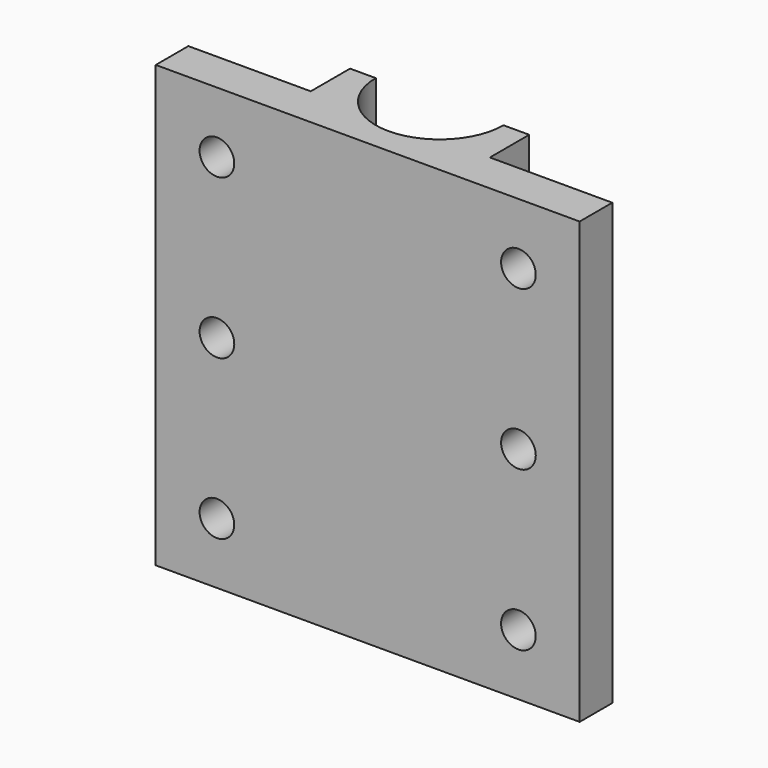
from build123d import *

# Parameters (mm, degrees)
F0_R      = 4.75
F1_DEPTH  = 7.5
F2_R      = 2.125
F3_DEPTH  = 25
F4_R      = 7.825
F5_DEPTH  = 5
F6_SIZE   = 2.5
F8_DEPTH  = 19.5
F9_R      = 2.125
F10_DEPTH = 25


# Not quite as in the source:
# - a pattern or mirror of a feature is missing from the dataset's text; its kind, count and spacing are read off the source's solid


with BuildPart() as f1:
    # F0 (on Top) → F1 (new body, symmetric)
    with BuildSketch(Plane.XY):
        with BuildLine():
            Line((-25.9795548635, -11.025), (0, -11.025))
            Line((0, -11.025), (25.9795548635, -11.025))
            Line((25.9795548635, -11.025), (25.9795548635, -6.025))
            Line((25.9795548635, -6.025), (10.9795548635, -6.025))
            Line((10.9795548635, -6.025), (10.9795548635, 1))
            ThreePointArc((10.9795548635, 1), (7.4338961857, 8.1417327701), (0, 11.025))
            ThreePointArc((0, 11.025), (-7.4338961857, 8.1417327701), (-10.9795548635, 1))
            Line((-10.9795548635, 1), (-10.9795548635, -6.025))
            Line((-10.9795548635, -6.025), (-25.9795548635, -6.025))
            Line((-25.9795548635, -6.025), (-25.9795548635, -11.025))
        make_face()
        Circle(F0_R, mode=Mode.SUBTRACT)
    extrude(amount=F1_DEPTH, both=True)

    # F2 (on face) → F3 (cut)
    with BuildSketch(Plane.XZ.offset(11.025)):
        with Locations((-18.4795548635, 0)):
            Circle(F2_R)
        with Locations((18.4795548635, 0)):
            Circle(F2_R)
    extrude(amount=-F3_DEPTH, mode=Mode.SUBTRACT)

    # F4 (on face) → F5 (cut)
    with BuildSketch(Plane.XY.offset(7.5)):
        Circle(F4_R)
    f5 = extrude(amount=-F5_DEPTH, mode=Mode.SUBTRACT)

    # F5_copies: F5 across plane
    add(f5.mirror(Plane(origin=(0, 0, 0), x_dir=(-1, 0, 0), z_dir=(0, 0, -1))), mode=Mode.SUBTRACT)

    # F6
    f6_edges = [f1.edges().sort_by_distance(p)[0] for p in [
        (-10.979555, -6.025, 0),
        (10.979555, -6.025, 0),
    ]]
    chamfer(f6_edges, length=F6_SIZE)

    # F7 (on face) → F8 (join)
    with BuildSketch(Plane.XY.offset(7.5)):
        with BuildLine():
            Line((-25.9795548635, -11.025), (0, -11.025))
            Line((0, -11.025), (25.9795548635, -11.025))
            Line((25.9795548635, -11.025), (25.9795548635, -6.025))
            Line((25.9795548635, -6.025), (10.9795548635, -6.025))
            Line((10.9795548635, -6.025), (10.9795548635, 0))
            Line((10.9795548635, 0), (7.825, 0))
            ThreePointArc((7.825, 0), (0, -7.825), (-7.825, 0))
            Line((-7.825, 0), (-10.9795548635, 0))
            Line((-10.9795548635, 0), (-10.9795548635, -6.025))
            Line((-10.9795548635, -6.025), (-25.9795548635, -6.025))
            Line((-25.9795548635, -6.025), (-25.9795548635, -11.025))
        make_face()
    f8 = extrude(amount=F8_DEPTH)

    # F8_copies: F8 across plane
    add(f8.mirror(Plane(origin=(0, 0, 0), x_dir=(-1, 0, 0), z_dir=(0, 0, -1))))

    # F9 (on face) → F10 (cut)
    with BuildSketch(Plane(origin=(0, -6.025, 0), x_dir=(-1, 0, 0), z_dir=(0, 1, 0))):
        with Locations((-18.4795548635, 19.5)):
            Circle(F9_R)
        with Locations((18.4795548635, 19.5)):
            Circle(F9_R)
    f10 = extrude(amount=-F10_DEPTH, mode=Mode.SUBTRACT)

    # F10_copies: F10 across plane
    add(f10.mirror(Plane(origin=(0, 0, 0), x_dir=(-1, 0, 0), z_dir=(0, 0, -1))), mode=Mode.SUBTRACT)


solid = f1.part
